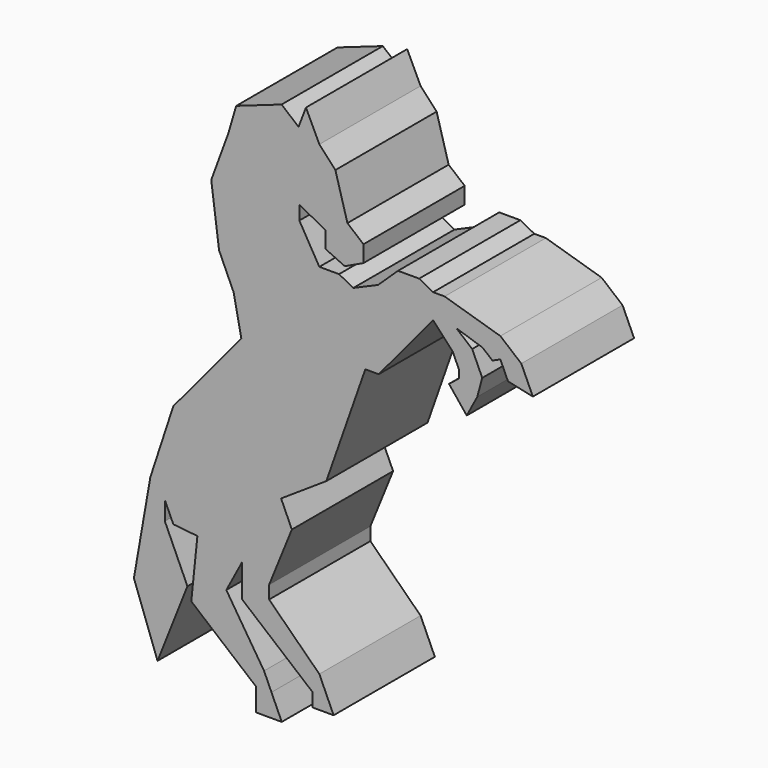
from build123d import *

# Parameters (mm, degrees)
F1_DEPTH = 25.4


# Not quite as in the source:
# - ends of sketch curves that miss each other by under 0.0002 mm in the source are joined


with BuildPart() as f1:
    # F0 (on Front) → F1 (new body)
    with BuildSketch(Plane.XZ):
        Polygon((0, 51.2815788388), (-2.6849012356, 56.9198653102), (-4.1696302487, 53.0196329049), (-7.5777377933, 55.8597221971), (-16.6846867651, 52.6580624282), (-18.2750094682, 47.2689494491), (-21.6973181814, 37.9454642534), (-20.1343216481, 26.0272607351), (-17.2047130764, 19.5402652025), (-15.6613234345, 11.8683064511), (-29.3124747088, -4.5130769722), (-33.9270979166, -18.5791757945), (-37.2212677423, -37.4857979189), (-32.480597056, -50.5585558089), (-26.4811083451, -35.4206826298), (-31.0107059295, -25.3908514852), (-31.0107059295, -21.6304793835), (-29.3124747088, -25.3908514852), (-24.4753230363, -25.888632983), (-25.7045285945, -37.8333391404), (-12.6969534904, -48.6729838072), (-12.6969534904, -53.2361328939), (-7.5467102784, -53.2361328939), (-9.6074856576, -48.6729838072), (-11.097422801, -45.3738346696), (-18.6685893591, -33.5405004938), (-15.5289131012, -27.6335775852), (-15.5289131012, -34.1437415194), (-1.3548218412, -45.9554828703), (-1.3548218412, -48.6729838072), (2.8690039134, -48.6729838072), (0, -42.3201844096), (-10.079539381, -32.4321724474), (-10.079539381, -29.8147555441), (-5.5140842237, -18.5791757945), (-7.6782507822, -13.7870889157), (1.4005823759, -7.7723623253), (9.2310756445, 14.5376751978), (11.9198445967, 14.5376751978), (22.8343526097, 27.6350863278), (26.7602472754, 23.3975637498), (28.004777182, 20.64181678), (28.004777182, 19.005872948), (26.0269176215, 17.4214001745), (29.5830273071, 12.9823932965), (31.7011885345, 16.9674586505), (32.6957959123, 20.64181678), (30.6835759384, 25.0974502414), (27.5022275746, 27.7485735714), (32.7634411399, 26.0272607351), (34.7447489485, 24.3761710855), (36.341868341, 25.0974502414), (37.8633029759, 21.7285566032), (42.8623110056, 20.64181678), (40.5427415461, 25.7263357936), (36.341868341, 29.2270630598), (25.148447603, 32.5854149557), (22.8343526097, 32.5854149557), (20.0345981866, 34.0735539794), (15.7886892557, 34.0735539794), (11.8005704135, 30.2826426923), (6.8094845357, 28.1176646778), (3.9549916983, 29.6348985285), (0, 29.6348985285), (-4.0098810568, 36.5146324039), (-4.0098810568, 39.3167249858), (1.2619188055, 36.5146324039), (1.2619188055, 33.1852734089), (5.1013175398, 31.4132459462), (8.8601689786, 33.1852734089), (8.8601689786, 36.5146324039), (5.6382901967, 39.1995310783), (3.2218813431, 47.7912090719), align=None)
    extrude(amount=F1_DEPTH)


solid = f1.part
